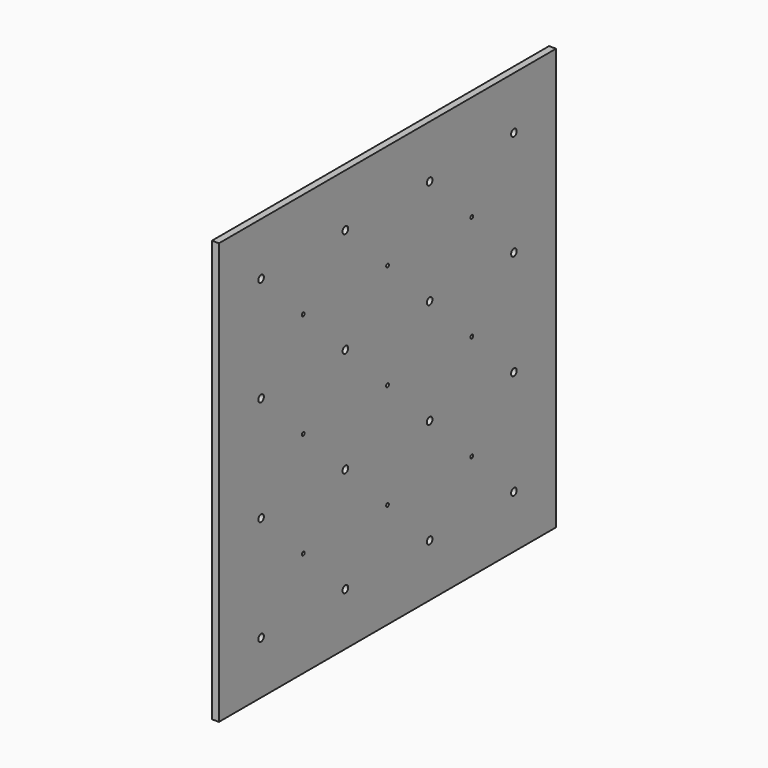
from build123d import *

# Parameters (mm, degrees)
F0_W     = 762
F0_H     = 762
F0_R     = 6.35
F0_R_2   = 3.175
F1_DEPTH = 12.7


# Not quite as in the source:
# - the program builds the solid bodies; features that only make, move or delete a surface that nothing else refers to are left out


with BuildPart() as f1:
    # F0 (on Right) → F1 (new body)
    with BuildSketch(Plane.YZ):
        with Locations((0, -33.2914479926)):
            Rectangle(F0_W, F0_H)
        with Locations((-285.75, -319.0414479926)):
            Circle(F0_R, mode=Mode.SUBTRACT)
        with Locations((-95.25, -319.0414479926)):
            Circle(F0_R, mode=Mode.SUBTRACT)
        with Locations((-285.75, -128.5414479926)):
            Circle(F0_R, mode=Mode.SUBTRACT)
        with Locations((-190.5, -223.7914479926)):
            Circle(F0_R_2, mode=Mode.SUBTRACT)
        with Locations((-95.25, -128.5414479926)):
            Circle(F0_R, mode=Mode.SUBTRACT)
        with Locations((95.25, -319.0414479926)):
            Circle(F0_R, mode=Mode.SUBTRACT)
        with Locations((285.75, -319.0414479926)):
            Circle(F0_R, mode=Mode.SUBTRACT)
        with Locations((0, -223.7914479926)):
            Circle(F0_R_2, mode=Mode.SUBTRACT)
        with Locations((95.25, -128.5414479926)):
            Circle(F0_R, mode=Mode.SUBTRACT)
        with Locations((190.5, -223.7914479926)):
            Circle(F0_R_2, mode=Mode.SUBTRACT)
        with Locations((285.75, -128.5414479926)):
            Circle(F0_R, mode=Mode.SUBTRACT)
        with Locations((-285.75, 61.9585520074)):
            Circle(F0_R, mode=Mode.SUBTRACT)
        with Locations((-190.5, -33.2914479926)):
            Circle(F0_R_2, mode=Mode.SUBTRACT)
        with Locations((-95.25, 61.9585520074)):
            Circle(F0_R, mode=Mode.SUBTRACT)
        with Locations((-285.75, 252.4585520074)):
            Circle(F0_R, mode=Mode.SUBTRACT)
        with Locations((-190.5, 157.2085520074)):
            Circle(F0_R_2, mode=Mode.SUBTRACT)
        with Locations((-95.25, 252.4585520074)):
            Circle(F0_R, mode=Mode.SUBTRACT)
        with Locations((0, -33.2914479926)):
            Circle(F0_R_2, mode=Mode.SUBTRACT)
        with Locations((95.25, 61.9585520074)):
            Circle(F0_R, mode=Mode.SUBTRACT)
        with Locations((190.5, -33.2914479926)):
            Circle(F0_R_2, mode=Mode.SUBTRACT)
        with Locations((285.75, 61.9585520074)):
            Circle(F0_R, mode=Mode.SUBTRACT)
        with Locations((0, 157.2085520074)):
            Circle(F0_R_2, mode=Mode.SUBTRACT)
        with Locations((95.25, 252.4585520074)):
            Circle(F0_R, mode=Mode.SUBTRACT)
        with Locations((190.5, 157.2085520074)):
            Circle(F0_R_2, mode=Mode.SUBTRACT)
        with Locations((285.75, 252.4585520074)):
            Circle(F0_R, mode=Mode.SUBTRACT)
    extrude(amount=F1_DEPTH)


solid = f1.part
